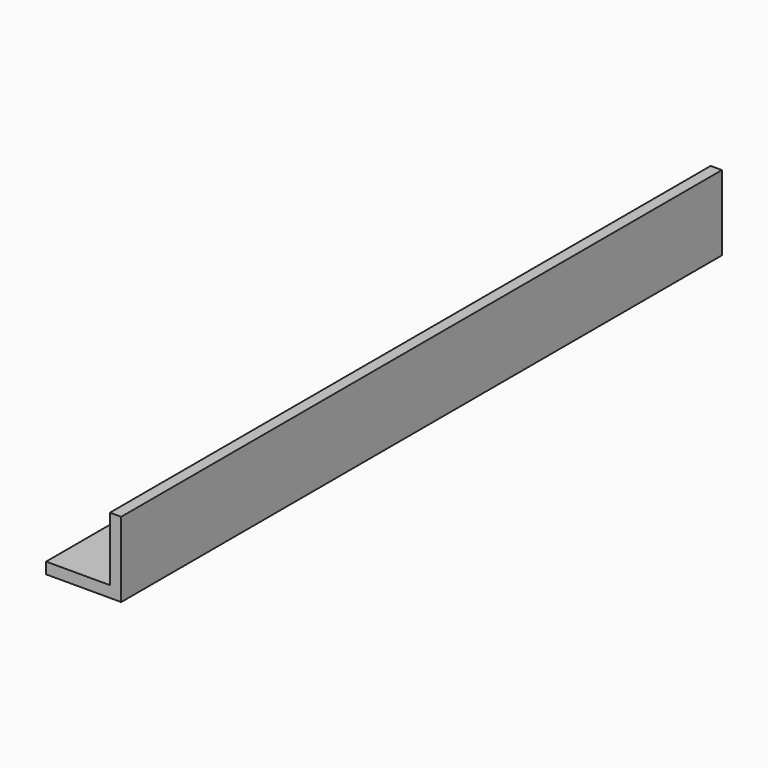
from build123d import *

# Parameters (mm, degrees)
F1_DEPTH = 100
F2_ANGLE = -45


with BuildPart() as f1:
    # F0 (on Front) → F1 (new body, symmetric)
    with BuildSketch(Plane.XZ):
        Polygon((-48.5120603115, 5.8607518886), (-50.6333806551, 3.739431545), (-36.4912450314, -10.4027040787), (-22.3491094076, 3.739431545), (-24.4704297512, 5.8607518886), (-36.4912450314, -6.1600633916), align=None)
    extrude(amount=F1_DEPTH, both=True)


with BuildPart() as f1_1:
    # F2: moved
    add(f1.part.rotate(Axis((-36.4912450314, 0, -10.4027040787), (0, 1, 0)), F2_ANGLE))


solid = f1_1.part
